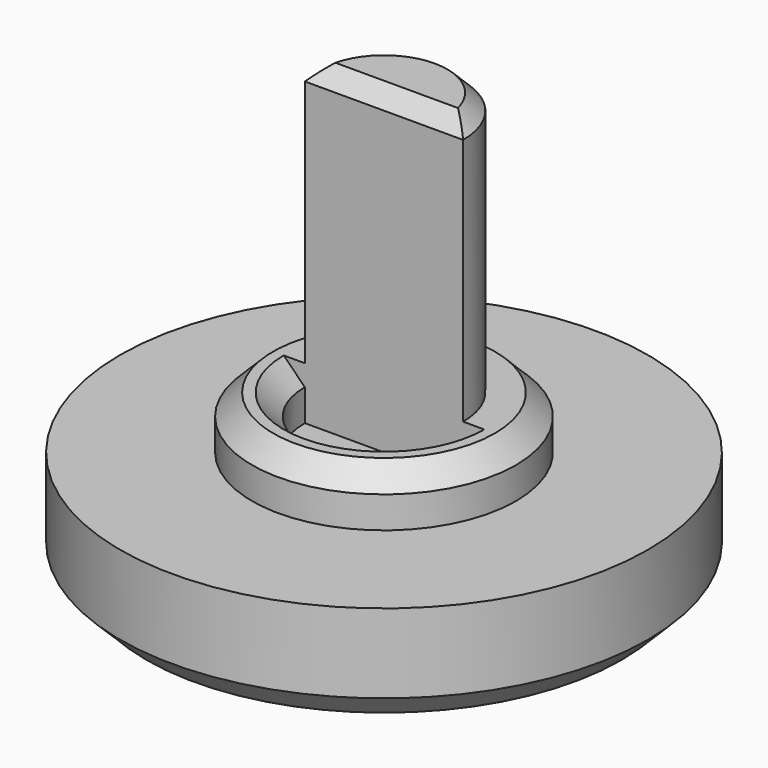
from build123d import *

# Parameters (mm, degrees)
F2_DEPTH = 8
F1_R     = 2.5
F4_DEPTH = 3
F1_R_2   = 5
F6_DEPTH = 2
F7_DEPTH = 2
F8_SIZE  = 0.4
F9_SIZE  = 0.3
F10_SIZE = 0.5
F11_SIZE = 0.4


with BuildPart() as f2:
    # F1 (on Top) → F2 (new body)
    with BuildSketch(Plane.XY):
        with BuildLine():
            Line((-1.5, 0), (1.5, 0))
            ThreePointArc((1.5, 0), (0, 1.5), (-1.5, 0))
        make_face()
    extrude(amount=F2_DEPTH)

    # F1 (on Top) → F4 (join)
    with BuildSketch(Plane.XY):
        Circle(F1_R)
        with BuildLine():
            ThreePointArc((-1.5, 0), (0, 1.5), (1.5, 0))
            ThreePointArc((1.5, 0), (0, -1.5), (-1.5, 0))
        make_face(mode=Mode.SUBTRACT)
    extrude(amount=F4_DEPTH)

    # F1 (on Top) → F6 (join)
    with BuildSketch(Plane.XY):
        Circle(F1_R_2)
        Circle(F1_R, mode=Mode.SUBTRACT)
    extrude(amount=F6_DEPTH)

    # F1 (on Top) → F7 (join)
    with BuildSketch(Plane.XY):
        with BuildLine():
            ThreePointArc((-1.5, 0), (0, -1.5), (1.5, 0))
            Line((1.5, 0), (-1.5, 0))
        make_face()
    extrude(amount=F7_DEPTH)

    # F8
    f8_edges = [f2.edges().sort_by_distance(p)[0] for p in [
        (-2.5, 0, 3),
    ]]
    chamfer(f8_edges, length=F8_SIZE)

    # F9
    f9_edges = [f2.edges().sort_by_distance(p)[0] for p in [
        (0, 1.5, 8),
        (0, 0, 8),
    ]]
    chamfer(f9_edges, length=F9_SIZE)

    # F10
    f10_edges = [f2.edges().sort_by_distance(p)[0] for p in [
        (-5, 0, 0),
    ]]
    chamfer(f10_edges, length=F10_SIZE)

    # F11
    f11_edges = [f2.edges().sort_by_distance(p)[0] for p in [
        (0, -1.5, 3),
    ]]
    chamfer(f11_edges, length=F11_SIZE)


solid = f2.part
